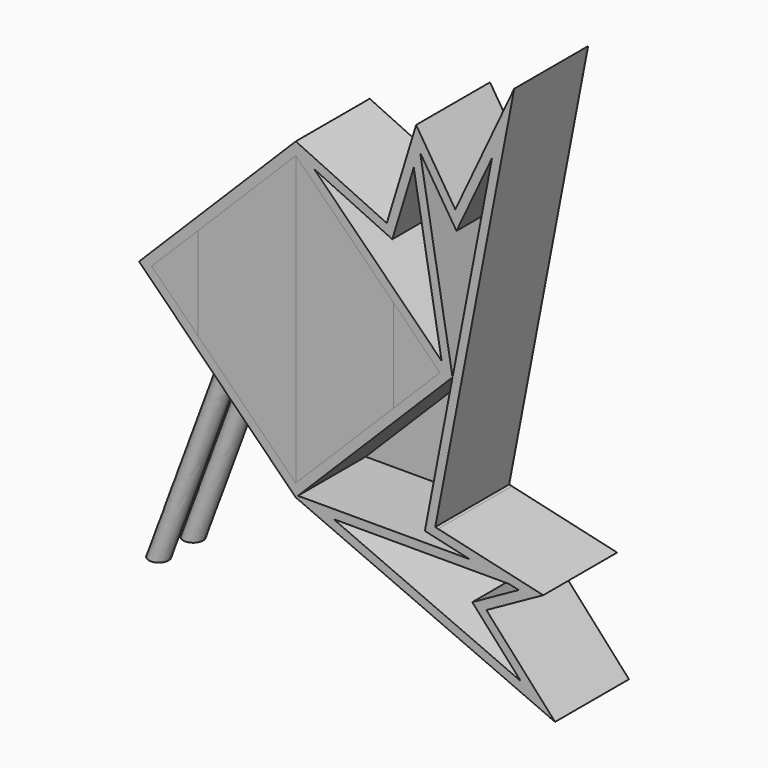
from build123d import *

# Parameters (mm, degrees)
F1_DEPTH  = 300
F3_DEPTH  = 300.001
F5_DEPTH  = 29
F6_W      = 114.4185625017
F6_H      = 85.1782578975
F7_DEPTH  = 787.3392
F8_R      = 32
F11_DEPTH = 29
F13_DEPTH = 1133
F16_DEPTH = 25
F18_DEPTH = 271


# Not quite as in the source:
# - ends of sketch curves that miss each other by under 0.0002 mm in the source are joined


with BuildPart() as f1:
    # F0 (on Front) → F1 (new body)
    with BuildSketch(Plane.XZ):
        Polygon((-21.1578859129, 461.1000678804), (-316.6142244869, 598.8736212078), (-256.6584088585, 538.9178055795), (-3.1787667582, 420.7183072818), (66.3378061044, 648.0967762461), (156.9029738247, 125.3564228963), (192.5026579675, 89.7567387535), (102.4632774249, -379.6587024434), (248.7953454256, -413.3447998695), (-310.5988806554, -413.3447998695), (-316.6142244868, -419.3601437008), (525.4976853374, -787.3391258891), (302.487393405, -539.9754328116), (487.1423766473, -437.4670079686), (145.604754854, -358.8439845974), (136.3912729242, -356.7230123856), (392.7879601275, 979.987250609), (201.4411428648, 572.4630155265), (74.1552898267, 772.8554183243), align=None)
        Polygon((379.9683977473, -442.5537108722), (407.0146211055, -448.7798356546), (256.5361856193, -532.3156662273), (413.9925393712, -706.9667319925), (-191.1109175542, -442.5537108722), align=None, mode=Mode.SUBTRACT)
        Polygon((320.7380442272, 758.304990145), (192.5026579675, 89.7567387535), (87.0405885007, 698.4817279892), (205.2598565448, 512.363297583), align=None, mode=Mode.SUBTRACT)
        Polygon((-316.6142244869, 598.8736212078), (-825.7311069412, 89.7567387535), (-588.7256799965, -147.2486881911), (-588.1432284625, -147.8311397252), (-316.6142244868, -419.3601437008), (-310.5988806554, -413.3447998695), (-301.6208118268, -404.3667310409), (192.5026579675, 89.7567387535), (156.9029738247, 125.3564228963), (-256.6584088585, 538.9178055795), align=None)
        Polygon((-316.6142244867, -378.347950392), (-577.6435249243, -117.3186499544), (-784.7189136323, 89.7567387535), (-316.6142244868, 557.861427899), (151.4904646587, 89.7567387535), align=None, mode=Mode.SUBTRACT)
        Polygon((-784.7189136323, 89.7567387535), (-577.6435249243, -117.3186499544), (-316.6142244867, -378.347950392), (151.4904646587, 89.7567387535), (-316.6142244868, 557.861427899), align=None)
        Polygon((87.0405885007, 698.4817279892), (192.5026579675, 89.7567387535), (320.7380442272, 758.304990145), (205.2598565448, 512.363297583), align=None)
        Polygon((256.5361856193, -532.3156662273), (407.0146211055, -448.7798356546), (379.9683977473, -442.5537108722), (-191.1109175542, -442.5537108722), (413.9925393712, -706.9667319925), align=None)
        Polygon((102.4632774249, -379.6587024434), (192.5026579675, 89.7567387535), (-301.6208118268, -404.3667310409), (-310.5988806554, -413.3447998695), (248.7953454256, -413.3447998695), align=None)
        Polygon((-3.1787667582, 420.7183072818), (-256.6584088585, 538.9178055795), (156.9029738247, 125.3564228963), (66.3378074545, 648.0967806623), align=None)
    extrude(amount=F1_DEPTH)

    # F2 (on face) → F3 (cut, through all)
    with BuildSketch(Plane.XZ.offset(300)):
        Polygon((-316.6142244869, 557.861427899), (-784.7189136323, 89.7567387535), (-316.6142244868, -378.347950392), (151.4904646587, 89.7567387536), align=None)
        Polygon((66.5084501228, 648.6549276806), (-3.1787679861, 420.7183078543), (-256.6584088585, 538.9178055795), (156.843021512, 125.4326254129), align=None)
        Polygon((205.2598565448, 512.363297583), (87.4447238518, 697.845477753), (192.441997649, 89.6960784351), (-309.5687277895, -412.3146470034), (248.6102088079, -412.3146470034), (102.6446876949, -378.7129298117), (320.7380442272, 758.304990145), align=None)
        Polygon((375.5810214862, -441.3146470034), (-193.9464883107, -441.3146470034), (413.9925393712, -706.9667319925), (256.5361856193, -532.3156662273), (407.306312324, -448.6179076805), align=None)
    extrude(amount=-F3_DEPTH, mode=Mode.SUBTRACT)


with BuildPart() as f5:
    # F4 (on face) → F5 (new body)
    with BuildSketch(Plane.XZ.offset(300)):
        Polygon((-316.6142244869, -378.347950392), (-316.6142244869, 557.861427899), (-634.7160485409, 239.7596038449), (-634.7160485409, -60.2461263379), align=None)
    extrude(amount=-F5_DEPTH)


with BuildPart() as f5b:
    # F4 (on face) → F5, piece 2 (new body)
    with BuildSketch(Plane.XZ.offset(300)):
        Polygon((151.4904646587, 89.7567387536), (0, 241.2472034122), (1.4904232565, -60.2433026486), align=None)
    extrude(amount=-F5_DEPTH)


with BuildPart() as f7:
    # F6 (on Top) → F7 (new body)
    with BuildSketch(Plane.XY):
        with Locations((468.2884040865, 458.3749382247)):
            Rectangle(F6_W, F6_H)
    extrude(amount=-F7_DEPTH)


with BuildPart() as f9:
    # F9: sweep along a path in F0
    with BuildLine(Plane.XZ) as f9_path:
        Line((-566.2141442299, -86.4508450031), (-825.7311069412, -787.3391258892))
    # F8 (on face) → F9 (sweep)
    with BuildSketch(Plane(origin=(0, 0, -787.3392), x_dir=(1, 0, 0), z_dir=(0, 0, -1))):
        with Locations((-825.7311069411, 220)):
            Circle(F8_R)
        with Locations((-825.7311069411, 80)):
            Circle(F8_R)
    sweep(path=f9_path.line)


with BuildPart() as f11:
    # F4 (on face) → F11 (new body)
    with BuildSketch(Plane.XZ.offset(300)):
        Polygon((-634.7160485409, -60.2461263379), (-634.7160485409, 239.7596038449), (-784.7189136323, 89.7567387535), align=None)
    extrude(amount=-F11_DEPTH)


with BuildPart() as f11b:
    # F4 (on face) → F11, piece 2 (new body)
    with BuildSketch(Plane.XZ.offset(300)):
        Polygon((0, 241.2472034122), (-316.6142244869, 557.861427899), (-316.6142244869, -378.347950392), (1.4904232565, -60.2433026486), align=None)
    extrude(amount=-F11_DEPTH)


with BuildPart() as f13:
    # F12 (on face) → F13 (new body)
    with BuildSketch(Plane(origin=(0, 0, 0), x_dir=(-1, 0, 0), z_dir=(0, 1, 0))):
        Polygon((444.9293017387, 0), (514.3381191953, -221.6362489923), (704.6059726342, -31.3683955535), align=None)
    extrude(amount=-F13_DEPTH)


with BuildPart() as f9_1:
    add(f9.part)

    # F14: cut F13
    add(f13.part, mode=Mode.SUBTRACT)


with BuildPart() as f16:
    # F15 (on face) → F16 (new body)
    with BuildSketch(Plane(origin=(0, 0, 0), x_dir=(-1, 0, 0), z_dir=(0, 1, 0))):
        Polygon((784.7189136323, 89.7567387535), (316.6142244869, 557.861427899), (-151.4904646587, 89.7567387536), (316.6142244868, -378.347950392), align=None)
    extrude(amount=-F16_DEPTH)


with BuildPart() as f16b:
    # F15 (on face) → F16, piece 2 (new body)
    with BuildSketch(Plane(origin=(0, 0, 0), x_dir=(-1, 0, 0), z_dir=(0, 1, 0))):
        Polygon((-248.6102088079, -412.3146470034), (309.5687277895, -412.3146470034), (-192.441997649, 89.6960784351), (-87.4447238518, 697.845477753), (-205.2598565448, 512.363297583), (-320.7380442272, 758.304990145), (-102.6446876949, -378.7129298117), align=None)
    extrude(amount=-F16_DEPTH)


with BuildPart() as f16c:
    # F15 (on face) → F16, piece 3 (new body)
    with BuildSketch(Plane(origin=(0, 0, 0), x_dir=(-1, 0, 0), z_dir=(0, 1, 0))):
        Polygon((-375.5810214862, -441.3146470034), (-407.306312324, -448.6179076805), (-256.5361856193, -532.3156662273), (-413.9925393712, -706.9667319925), (193.9464883107, -441.3146470034), align=None)
    extrude(amount=-F16_DEPTH)


with BuildPart() as f16d:
    # F15 (on face) → F16, piece 4 (new body)
    with BuildSketch(Plane(origin=(0, 0, 0), x_dir=(-1, 0, 0), z_dir=(0, 1, 0))):
        Polygon((3.1787679861, 420.7183078543), (-66.5084501228, 648.6549276806), (-156.843021512, 125.4326254129), (256.6584088585, 538.9178055795), align=None)
    extrude(amount=-F16_DEPTH)


with BuildPart() as f18:
    # F17 (on face) → F18 (new body)
    with BuildSketch(Plane(origin=(0, 0, 0), x_dir=(-1, 0, 0), z_dir=(0, 1, 0))):
        Polygon((111.5618799141, 352.8090833263), (82.5618799141, 323.8090833263), (550.6665690596, 323.8090833263), (521.6665690596, 352.8090833263), align=None)
    extrude(amount=-F18_DEPTH)


with BuildPart() as f18b:
    # F17 (on face) → F18, piece 2 (new body)
    with BuildSketch(Plane(origin=(0, 0, 0), x_dir=(-1, 0, 0), z_dir=(0, 1, 0))):
        Polygon((-136.9904646587, 104.2567387535), (-151.4904646587, 89.7567387536), (-136.9904646586, 75.2567387535), (770.2189136323, 75.2567387535), (784.7189136323, 89.7567387535), (770.2189136323, 104.2567387535), align=None)
    extrude(amount=-F18_DEPTH)


with BuildPart() as f18c:
    # F17 (on face) → F18, piece 3 (new body)
    with BuildSketch(Plane(origin=(0, 0, 0), x_dir=(-1, 0, 0), z_dir=(0, 1, 0))):
        Polygon((550.6665690596, -144.2956058192), (82.5618799141, -144.2956058192), (111.5618799141, -173.2956058192), (521.6665690596, -173.2956058192), align=None)
    extrude(amount=-F18_DEPTH)


solid = Compound([f1.part, f5.part, f5b.part, f11.part, f11b.part, f9_1.part, f16.part, f16b.part, f16c.part, f16d.part, f18.part, f18b.part, f18c.part])
